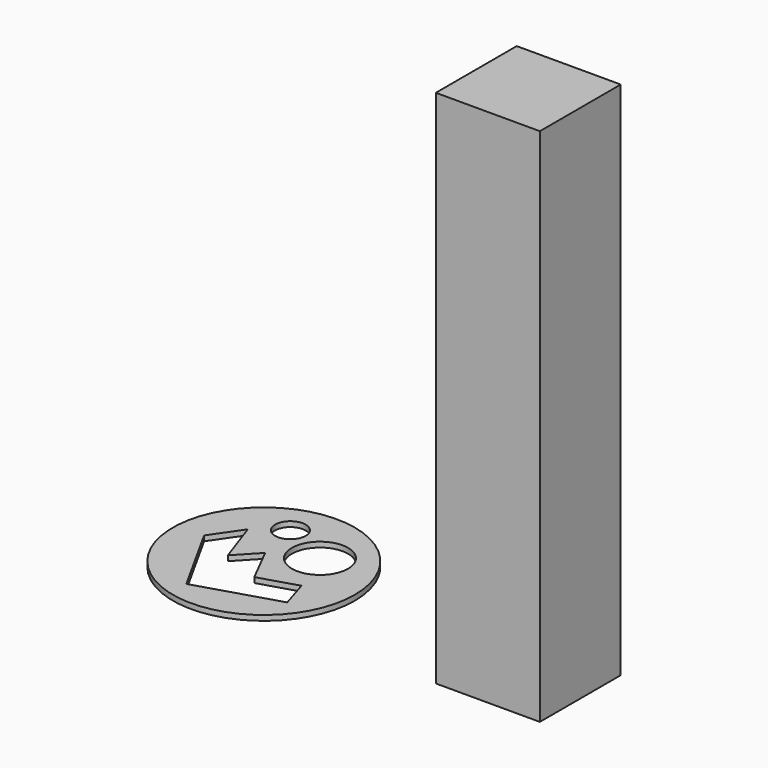
from build123d import *

# Parameters (mm, degrees)
F0_W     = 19.9999965323
F0_H     = 19.4392482125
F0_W_2   = 18.7999965323
F0_H_2   = 18.2392482125
F1_DEPTH = 100
F0_R     = 17.5
F0_R_2   = 5.4162553958
F0_R_3   = 2.9408408329
F2_DEPTH = 1


with BuildPart() as f1:
    # F0 (on Top) → F1 (new body)
    with BuildSketch(Plane.XY):
        with Locations((1.7338e-06, 0.2803758938)):
            Rectangle(F0_W, F0_H)
        with Locations((1.7338e-06, 0.2803758938)):
            Rectangle(F0_W_2, F0_H_2, mode=Mode.SUBTRACT)
        with Locations((1.7338e-06, 0.2803758938)):
            Rectangle(F0_W_2, F0_H_2)
    extrude(amount=F1_DEPTH)


with BuildPart() as f2:
    # F0 (on Top) → F2 (new body)
    with BuildSketch(Plane.XY):
        with Locations((-53.8173690438, 3.9858361706)):
            Circle(F0_R)
        Polygon((-58.2814313382, -9.0601613548), (-66.0512670875, 4.926905036), (-62.169354409, 10.5733172968), (-59.2285133898, 2.1036986727), (-55.3466044366, 6.2208748423), (-51.6999661922, -0.9547745576), (-44.4066822529, 1.2802636484), (-42.7010375303, -4.2855254412), align=None, mode=Mode.SUBTRACT)
        with Locations((-47.8180535138, 9.9851489067)):
            Circle(F0_R_2, mode=Mode.SUBTRACT)
        with Locations((-56.9934770465, 14.3375927582)):
            Circle(F0_R_3, mode=Mode.SUBTRACT)
    extrude(amount=F2_DEPTH)


solid = Compound([f1.part, f2.part])
